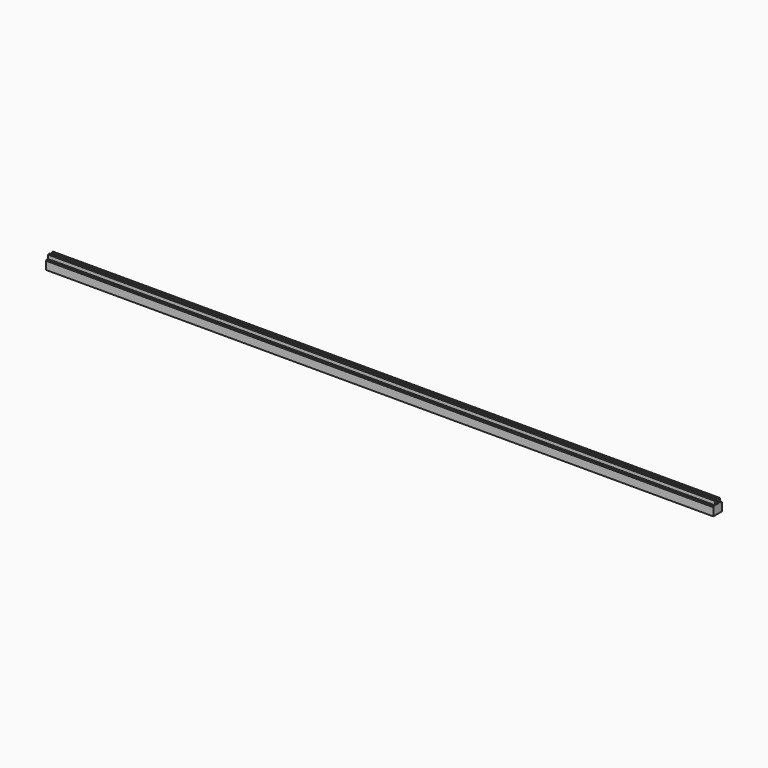
from build123d import *

# Parameters (mm, degrees)
F1_W     = 40
F1_H     = 19
F3_DEPTH = 1275
F2_W     = 80
F2_H     = 100
F4_DEPTH = 25
F6_DEPTH = 40


with BuildPart() as f3:
    # F1 (on Right) → F3 (new body, symmetric)
    with BuildSketch(Plane.YZ):
        Polygon((20, 33), (20, 63), (17, 66), (12, 66), (12, 80), (4, 80), (4, 66), (-4, 66), (-4, 80), (-12, 80), (-12, 66), (-17, 66), (-20, 63), (-20, 33), align=None)
        with Locations((0, 23.5)):
            Rectangle(F1_W, F1_H)
    extrude(amount=F3_DEPTH, both=True)

    # F2 (on Front) → F4 (cut, symmetric)
    with BuildSketch(Plane.XZ):
        with Locations((-1275, 83)):
            Rectangle(F2_W, F2_H)
        with Locations((-1275, -83)):
            Rectangle(F2_W, F2_H)
        with Locations((1275, 83)):
            Rectangle(F2_W, F2_H)
        with Locations((1275, -83)):
            Rectangle(F2_W, F2_H)
    extrude(amount=F4_DEPTH, both=True, mode=Mode.SUBTRACT)

    # F5 (on face) → F6 (cut, through all)
    with BuildSketch(Plane.XZ.offset(20)):
        Polygon((-1235, 33), (-1275, 33), (-1275, 14), (1275, 14), (1275, 33), (1235, 33), align=None)
    extrude(amount=-F6_DEPTH, mode=Mode.SUBTRACT)


solid = f3.part
